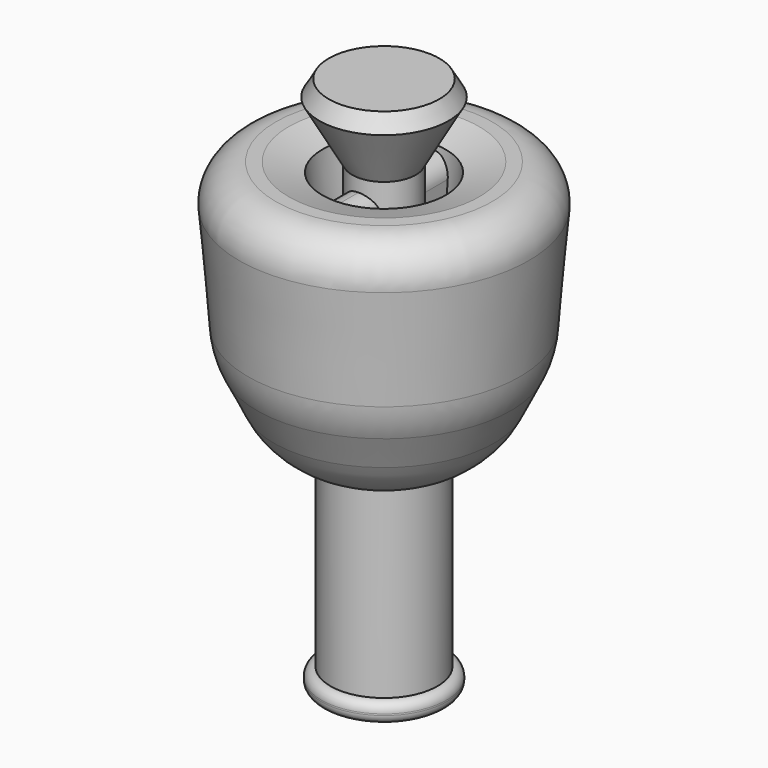
from build123d import *

# Parameters (mm, degrees)
F2_W     = 2
F2_H     = 3
F3_DEPTH = 5
F4_SIZE  = 0.99999
F5_R     = 0.99999
F6_R     = 2
F7_SIZE  = 1
F8_R     = 5
F9_R     = 0.49999


# Not quite as in the source:
# - a fillet or chamfer is up to 0.001 mm smaller than in the source, because OpenCascade refuses the exact size


with BuildPart() as f1:
    # F0 (on Front) → F1 (revolve)
    with BuildSketch(Plane.XZ):
        Polygon((0, 14.5783070475), (0, 29.156614095), (-4, 29.156614095), (-1.7319330946, 25.1257959753), (-1.7319330946, 22.7402094752), (-1.7319330946, 19.5320062339), align=None)
    revolve(axis=Axis((0, 0, 14.5783070475), (0, 0, -1)))

    # F7
    f7_edges = [f1.edges().sort_by_distance(p)[0] for p in [
        (4, 0, 29.156614),
    ]]
    chamfer(f7_edges, length=F7_SIZE)


with BuildPart() as f1b:
    # F0 (on Front) → F1, piece 2 (revolve)
    with BuildSketch(Plane.XZ):
        Polygon((-3.3527006079, 24.6845433628), (-5.1671702769, 25.1912331348), (-8.0463260766, 25.1912331348), (-7.306943031, 16.3838422066), (-5.1270102505, 11.9417147851), (-2.9059470054, 11.0779680451), (-2.9059470054, 1.0779680451), (-3.4059470054, 1.0779680451), (-3.4059470054, 0), (-3, 0), (-1.6558364648, 0), (-1.6558364648, 11.0725850007), (-2.7111049439, 17.0419772207), align=None)
    revolve(axis=Axis((0, 0, 14.5783070475), (0, 0, -1)))

    # F6
    f6_edges = [f1b.edges().sort_by_distance(p)[0] for p in [
        (8.046326, 0, 25.191233),
    ]]
    fillet(f6_edges, radius=F6_R)

    # F8
    f8_edges = [f1b.edges().sort_by_distance(p)[0] for p in [
        (7.306943, 0, 16.383842),
        (5.12701, 0, 11.941715),
    ]]
    fillet(f8_edges, radius=F8_R)

    # F9 (radius 0.5 in the source; OpenCascade refuses exactly that, so slightly less here)
    f9_edges = [f1b.edges().sort_by_distance(p)[0] for p in [
        (3.405947, 0, 0),
        (3.405947, 0, 1.077968),
    ]]
    fillet(f9_edges, radius=F9_R)


with BuildPart() as f3:
    # F2 (on Front) → F3 (new body, symmetric)
    with BuildSketch(Plane.XZ):
        with Locations((0, 22.9238849133)):
            Rectangle(F2_W, F2_H)
    extrude(amount=F3_DEPTH, both=True)

    # F4 (size 1 in the source; OpenCascade refuses exactly that, so slightly less here)
    f4_edges = [f3.edges().sort_by_distance(p)[0] for p in [
        (-1, 0, 21.423885),
        (1, 0, 21.423885),
    ]]
    chamfer(f4_edges, length=F4_SIZE)

    # F5 (radius 1 in the source; OpenCascade refuses exactly that, so slightly less here)
    f5_edges = [f3.edges().sort_by_distance(p)[0] for p in [
        (-1, 0, 24.423885),
        (1, 0, 24.423885),
    ]]
    fillet(f5_edges, radius=F5_R)


solid = Compound([f1.part, f1b.part, f3.part])
